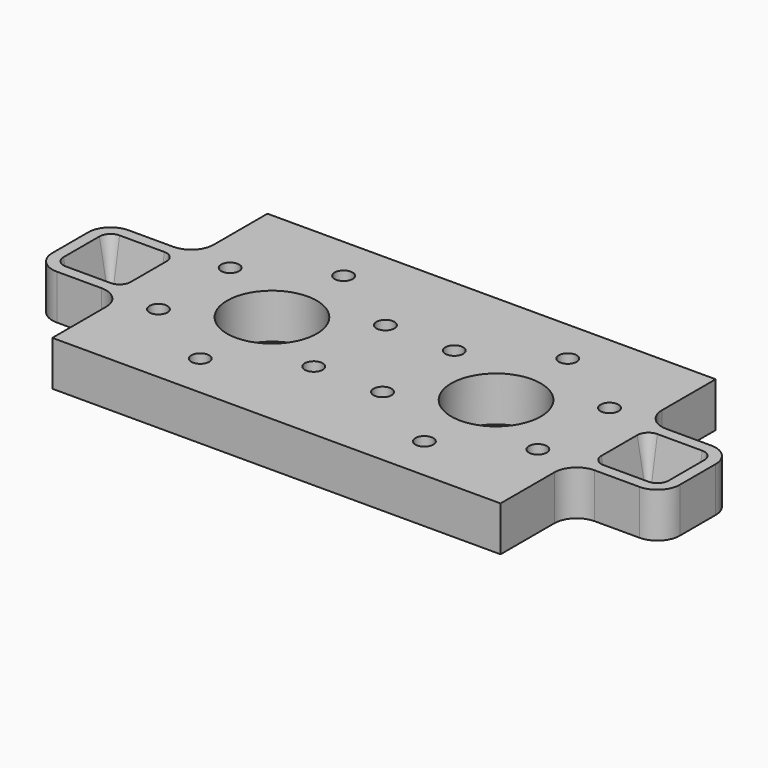
from build123d import *

# Parameters (mm, degrees)
F0_W            = 50.8
F0_H            = 50.8
F0_R            = 25.4
F1_DEPTH        = 25.4
F2_R            = 12.7
F4_D            = 10.16
F4_COPIES_COUNT = 6
F5_DEPTH        = 25.401
F5_TAPER        = 10


# Not quite as in the source:
# - a pattern or mirror of a feature is missing from the dataset's text; its kind, count and spacing are read off the source's solid


with BuildPart() as f1:
    # F0 (on Top) → F1 (new body)
    with BuildSketch(Plane.XY):
        with Locations((88.9, 0)):
            Rectangle(F0_W, F0_H)
        Polygon((63.5, 25.4), (63.5, 76.2), (-63.5, 76.2), (-63.5, -76.2), (63.5, -76.2), (63.5, -25.4), align=None)
        Circle(F0_R, mode=Mode.SUBTRACT)
    extrude(amount=F1_DEPTH)

    # F2
    f2_edges = [f1.edges().sort_by_distance(p)[0] for p in [
        (63.5, -25.4, 12.7),
        (63.5, 25.4, 12.7),
        (114.3, -25.4, 12.7),
        (114.3, 25.4, 12.7),
    ]]
    fillet(f2_edges, radius=F2_R)

    # F4 (through all)
    with Locations(Plane.XY.offset(25.4)):
        with Locations((0, -50.8)):
            f4 = Hole(F4_D / 2)

    # F4_copies: F4 ×6 about axis
    f4_copies_axis = Axis((0, 0, 0), (0, 0, 1))
    for i in range(1, F4_COPIES_COUNT):
        add(f4.rotate(f4_copies_axis, i * 360 / F4_COPIES_COUNT), mode=Mode.SUBTRACT)

    # F3 (on face) → F5 (cut, through all)
    with BuildSketch(Plane.XY.offset(25.4)):
        with BuildLine():
            ThreePointArc((107.9500002354, 12.7), (106.090128227, 17.190128227), (101.6, 19.0500002354))
            Line((101.6, 19.0500002354), (76.2000002354, 19.0500002354))
            ThreePointArc((76.2000002354, 19.0500002354), (71.7098721749, 17.190128296), (69.8500002354, 12.7000002354))
            Line((69.8500002354, 12.7000002354), (69.8500002354, -12.7000002354))
            ThreePointArc((69.8500002354, -12.7000002354), (71.7098721749, -17.190128296), (76.2000002354, -19.0500002354))
            Line((76.2000002354, -19.0500002354), (101.6, -19.0500002354))
            ThreePointArc((101.6, -19.0500002354), (106.090128227, -17.190128227), (107.9500002354, -12.7))
            Line((107.9500002354, -12.7), (107.9500002354, 12.7))
        make_face()
    extrude(amount=-F5_DEPTH, taper=F5_TAPER, mode=Mode.SUBTRACT)

    # F6: F1 across face


with BuildPart() as f1_1:
    add(f1.part)
    add(f1.part.mirror(Plane(origin=(-63.5, 0, 12.7), x_dir=(0, -1, 0), z_dir=(-1, 0, 0))))


solid = f1_1.part
